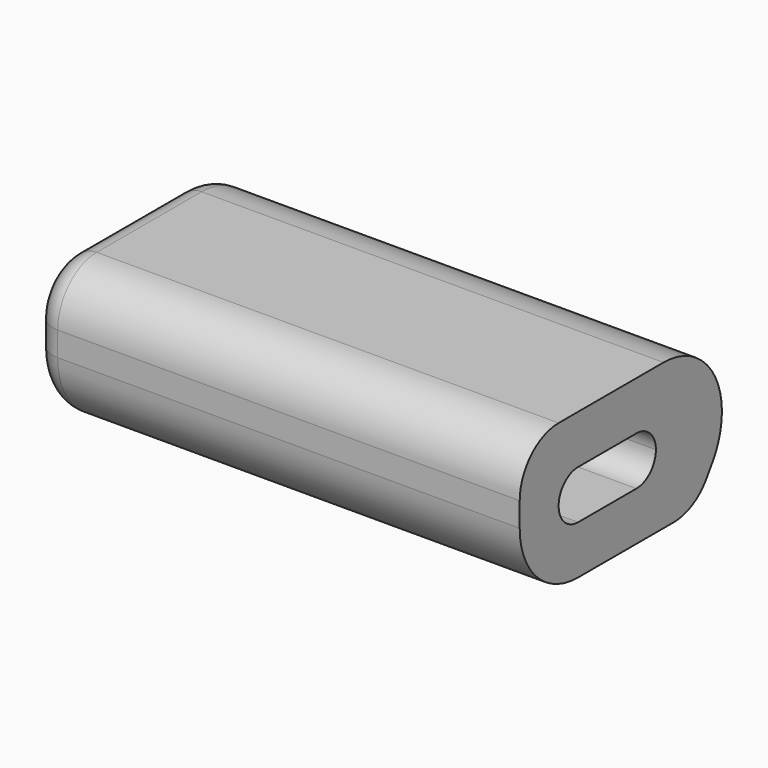
from build123d import *

# Parameters (mm, degrees)
F1_DEPTH = 100
F2_R     = 15
F3_W     = 25
F3_H     = 10
F4_DEPTH = 80
F5_R     = 4.99999
F6_R     = 10
F7_R     = 5


# Not quite as in the source:
# - a fillet or chamfer is up to 0.001 mm smaller than in the source, because OpenCascade refuses the exact size


with BuildPart() as f1:
    # F0 (on Right) → F1 (new body)
    with BuildSketch(Plane.YZ):
        Polygon((65, 0), (0, 0), (0, -30), (45, -30), align=None)
    extrude(amount=F1_DEPTH)

    # F2
    f2_edges = [f1.edges().sort_by_distance(p)[0] for p in [
        (50, 65, 0),
        (50, 0, -30),
    ]]
    fillet(f2_edges, radius=F2_R)

    # F3 (on face) → F4 (cut)
    with BuildSketch(Plane.YZ.offset(100)):
        with Locations((22.5, -15)):
            Rectangle(F3_W, F3_H)
    extrude(amount=-F4_DEPTH, mode=Mode.SUBTRACT)

    # F5 (radius 5 in the source; OpenCascade refuses exactly that, so slightly less here)
    f5_edges = [f1.edges().sort_by_distance(p)[0] for p in [
        (60, 10, -10),
        (60, 10, -20),
        (60, 35, -10),
        (60, 35, -20),
    ]]
    fillet(f5_edges, radius=F5_R)

    # F6
    f6_edges = [f1.edges().sort_by_distance(p)[0] for p in [
        (50, 0, 0),
        (50, 45, -30),
    ]]
    fillet(f6_edges, radius=F6_R)

    # F7
    f7_edges = [f1.edges().sort_by_distance(p)[0] for p in [
        (0, 23.486122, 0),
    ]]
    fillet(f7_edges, radius=F7_R)


solid = f1.part
